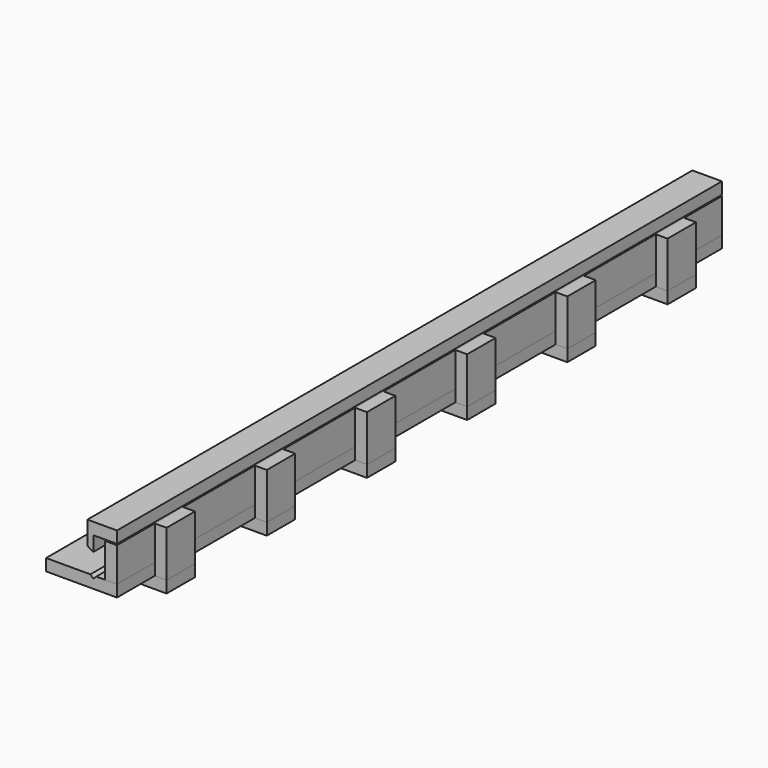
from build123d import *

# Parameters (mm, degrees)
F3_W      = 12.7
F3_H      = 36.83
F6_DEPTH  = 406.4
F7_DEPTH  = 406.4
F5_W      = 25.4
F5_H      = 12.7
F8_DEPTH  = 406.4
F9_W      = 38.1
F9_H      = 49.53
F10_DEPTH = 12.7
F11_W     = 38.1
F11_H     = 12.7
F12_DEPTH = 76.2


# Not quite as in the source:
# - a variable given as a bare number and used for a length is read in inches; the dataset says mm whatever the document's units were


with BuildPart() as f6:
    # F3 (on Front) → F6 (new body, symmetric)
    with BuildSketch(Plane.XZ):
        with Locations((6.35, 18.415)):
            Rectangle(F3_W, F3_H)
    extrude(amount=F6_DEPTH, both=True)


with BuildPart() as f7:
    # F4 (on Front) → F7 (new body, symmetric)
    with BuildSketch(Plane.XZ):
        Polygon((12.7, -12.7), (12.7, 0), (-9.525, 0), (-12.7, -3.175), (-15.875, 0), (-63.5, 0), (-63.5, -12.7), align=None)
    extrude(amount=F7_DEPTH, both=True)


with BuildPart() as f8:
    # F5 (on Front) → F8 (new body, symmetric)
    with BuildSketch(Plane.XZ):
        with Locations((0, 44.45)):
            Rectangle(F5_W, F5_H)
        Polygon((-12.7, 22.225), (-12.7, 38.1), (-12.7, 50.8), (-19.05, 50.8), (-19.05, 25.8911742094), align=None)
    extrude(amount=F8_DEPTH, both=True)


with BuildPart() as f10:
    # F9 (on face) → F10 (new body)
    with BuildSketch(Plane.YZ.offset(12.7)):
        with Locations((-336.55, 12.065)):
            Rectangle(F9_W, F9_H)
    extrude(amount=F10_DEPTH)


with BuildPart() as f10b:
    # F9 (on face) → F10, piece 2 (new body)
    with BuildSketch(Plane.YZ.offset(12.7)):
        with Locations((-201.93, 12.065)):
            Rectangle(F9_W, F9_H)
    extrude(amount=F10_DEPTH)


with BuildPart() as f10c:
    # F9 (on face) → F10, piece 3 (new body)
    with BuildSketch(Plane.YZ.offset(12.7)):
        with Locations((-67.31, 12.065)):
            Rectangle(F9_W, F9_H)
    extrude(amount=F10_DEPTH)


with BuildPart() as f10d:
    # F9 (on face) → F10, piece 4 (new body)
    with BuildSketch(Plane.YZ.offset(12.7)):
        with Locations((67.31, 12.065)):
            Rectangle(F9_W, F9_H)
    extrude(amount=F10_DEPTH)


with BuildPart() as f10e:
    # F9 (on face) → F10, piece 5 (new body)
    with BuildSketch(Plane.YZ.offset(12.7)):
        with Locations((201.93, 12.065)):
            Rectangle(F9_W, F9_H)
    extrude(amount=F10_DEPTH)


with BuildPart() as f10f:
    # F9 (on face) → F10, piece 6 (new body)
    with BuildSketch(Plane.YZ.offset(12.7)):
        with Locations((336.55, 12.065)):
            Rectangle(F9_W, F9_H)
    extrude(amount=F10_DEPTH)


with BuildPart() as f12:
    # F11 (on face) → F12 (new body)
    with BuildSketch(Plane.YZ.offset(25.4)):
        with Locations((-336.55, -19.05)):
            Rectangle(F11_W, F11_H)
    extrude(amount=-F12_DEPTH)


with BuildPart() as f12b:
    # F11 (on face) → F12, piece 2 (new body)
    with BuildSketch(Plane.YZ.offset(25.4)):
        with Locations((-201.93, -19.05)):
            Rectangle(F11_W, F11_H)
    extrude(amount=-F12_DEPTH)


with BuildPart() as f12c:
    # F11 (on face) → F12, piece 3 (new body)
    with BuildSketch(Plane.YZ.offset(25.4)):
        with Locations((-67.31, -19.05)):
            Rectangle(F11_W, F11_H)
    extrude(amount=-F12_DEPTH)


with BuildPart() as f12d:
    # F11 (on face) → F12, piece 4 (new body)
    with BuildSketch(Plane.YZ.offset(25.4)):
        with Locations((67.31, -19.05)):
            Rectangle(F11_W, F11_H)
    extrude(amount=-F12_DEPTH)


with BuildPart() as f12e:
    # F11 (on face) → F12, piece 5 (new body)
    with BuildSketch(Plane.YZ.offset(25.4)):
        with Locations((201.93, -19.05)):
            Rectangle(F11_W, F11_H)
    extrude(amount=-F12_DEPTH)


with BuildPart() as f12f:
    # F11 (on face) → F12, piece 6 (new body)
    with BuildSketch(Plane.YZ.offset(25.4)):
        with Locations((336.55, -19.05)):
            Rectangle(F11_W, F11_H)
    extrude(amount=-F12_DEPTH)


solid = Compound([f6.part, f7.part, f8.part, f10.part, f10b.part, f10c.part, f10d.part, f10e.part, f10f.part, f12.part, f12b.part, f12c.part, f12d.part, f12e.part, f12f.part])
